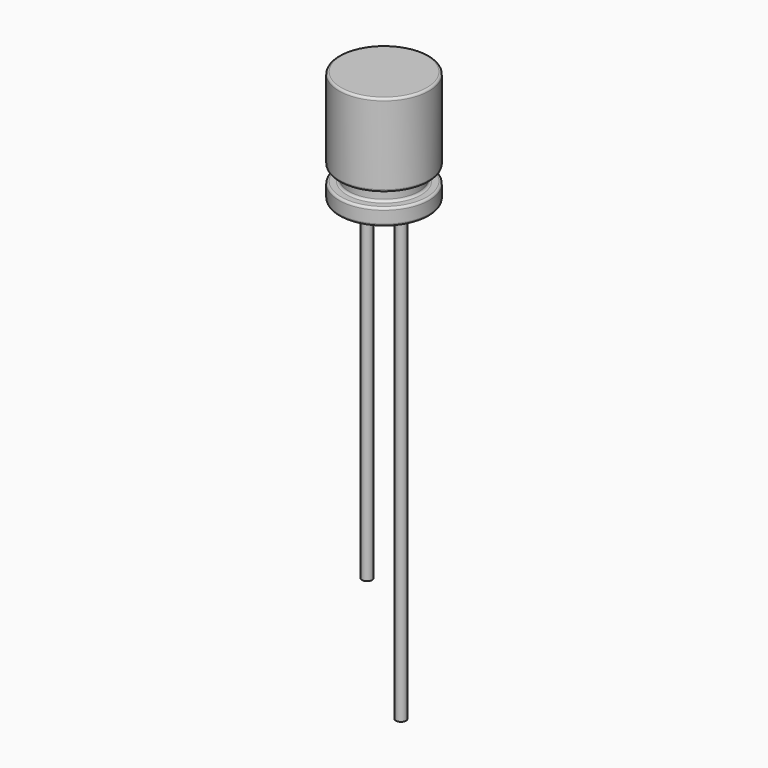
from build123d import *

# Parameters (mm, degrees)
F0_R     = 2
F1_DEPTH = 5
F2_W     = 1.057303627
F2_H     = 0.604173576
F4_R     = 0.1
F5_R     = 0.225
F6_DEPTH = 15
F7_DEPTH = 5


with BuildPart() as f1:
    # F0 (on Top) → F1 (new body)
    with BuildSketch(Plane.XY):
        Circle(F0_R)
    extrude(amount=F1_DEPTH)

    # F2 (on Front) → F3 (revolve, cut)
    with BuildSketch(Plane.XZ):
        with Locations((2.0760625484, 1.0352871905)):
            Rectangle(F2_W, F2_H)
    revolve(axis=Axis((0, 0, 0), (0, 0, 1)), mode=Mode.SUBTRACT)

    # F4
    f4_edges = [f1.edges().sort_by_distance(p)[0] for p in [
        (-2, 0, 1.337374),
        (-1.547411, 0, 1.337374),
        (-1.547411, 0, 0.7332),
        (-2, 0, 0.7332),
        (-2, 0, 5),
        (-2, 0, 0),
    ]]
    fillet(f4_edges, radius=F4_R)

    # F5 (on face) → F6 (join)
    with BuildSketch(Plane(origin=(0, 0, 0), x_dir=(1, 0, 0), z_dir=(0, 0, -1))):
        with Locations((-0.75, 0)):
            Circle(F5_R)
        with BuildLine():
            ThreePointArc((0.975, 0), (0.75, 0.225), (0.525, 0))
            ThreePointArc((0.525, 0), (0.75, -0.225), (0.975, 0))
        make_face()
    extrude(amount=F6_DEPTH)

    # F7 (add): a face of the model
    f7_faces = [f1.faces().sort_by_distance(p)[0] for p in [
        (0.75, 0, -15),
    ]]
    extrude(f7_faces, amount=F7_DEPTH)


solid = f1.part
